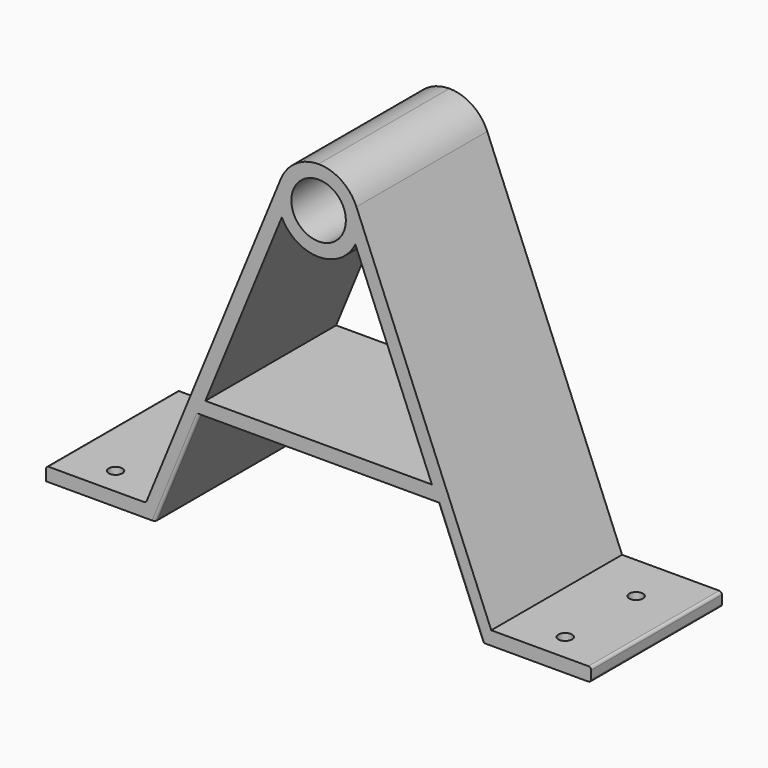
from build123d import *

# Parameters (mm, degrees)
F0_R     = 10
F1_DEPTH = 60
F2_R     = 2.5
F3_DEPTH = 5.001
F4_R     = 1


with BuildPart() as f1:
    # F0 (on Front) → F1 (new body)
    with BuildSketch(Plane.XZ):
        with BuildLine():
            ThreePointArc((86.1209118397, 120.6895440801), (85.0074372508, 114.5277053764), (86.5065387851, 108.4481678561))
            ThreePointArc((86.5065387851, 108.4481678561), (100, 100), (113.4934612149, 108.4481678561))
            ThreePointArc((113.4934612149, 108.4481678561), (114.9925627492, 114.5277053764), (113.8790881603, 120.6895440801))
            ThreePointArc((113.8790881603, 120.6895440801), (108.356340072, 127.4567885348), (100, 130))
            ThreePointArc((100, 130), (91.643659928, 127.4567885348), (86.1209118397, 120.6895440801))
        make_face()
        with Locations((100, 115)):
            Circle(F0_R, mode=Mode.SUBTRACT)
        with BuildLine():
            Line((58.4471400894, 40), (86.5065387851, 108.4481678561))
            ThreePointArc((86.5065387851, 108.4481678561), (85.0074372508, 114.5277053764), (86.1209118397, 120.6895440801))
            Line((86.1209118397, 120.6895440801), (36.6458690181, 0))
            Line((36.6458690181, 0), (0, 0))
            Line((0, 0), (0, -5))
            Line((0, -5), (40, -5))
            Line((40, -5), (56.3974578573, 35))
            Line((56.3974578573, 35), (143.6025421427, 35))
            Line((143.6025421427, 35), (160, -5))
            Line((160, -5), (200, -5))
            Line((200, -5), (200, 0))
            Line((200, 0), (163.3541309819, 0))
            Line((163.3541309819, 0), (113.8790881603, 120.6895440801))
            ThreePointArc((113.8790881603, 120.6895440801), (114.9925627492, 114.5277053764), (113.4934612149, 108.4481678561))
            Line((113.4934612149, 108.4481678561), (141.5528599106, 40))
            Line((141.5528599106, 40), (58.4471400894, 40))
        make_face()
    extrude(amount=-F1_DEPTH)

    # F2 (on face) → F3 (cut, through all)
    with BuildSketch(Plane.XY):
        with Locations((182.5, 10)):
            Circle(F2_R)
        with Locations((182.5, 42.5)):
            Circle(F2_R)
        with Locations((17.5, 10)):
            Circle(F2_R)
        with Locations((17.5, 42.5)):
            Circle(F2_R)
    extrude(amount=-F3_DEPTH, mode=Mode.SUBTRACT)

    # F4
    f4_edges = [f1.edges().sort_by_distance(p)[0] for p in [
        (200, 30, 0),
        (200, 30, -5),
        (0, 30, 0),
        (151.801271, 0, 15),
        (48.198729, 0, 15),
        (36.645869, 30, 0),
    ]]
    fillet(f4_edges, radius=F4_R)


solid = f1.part
